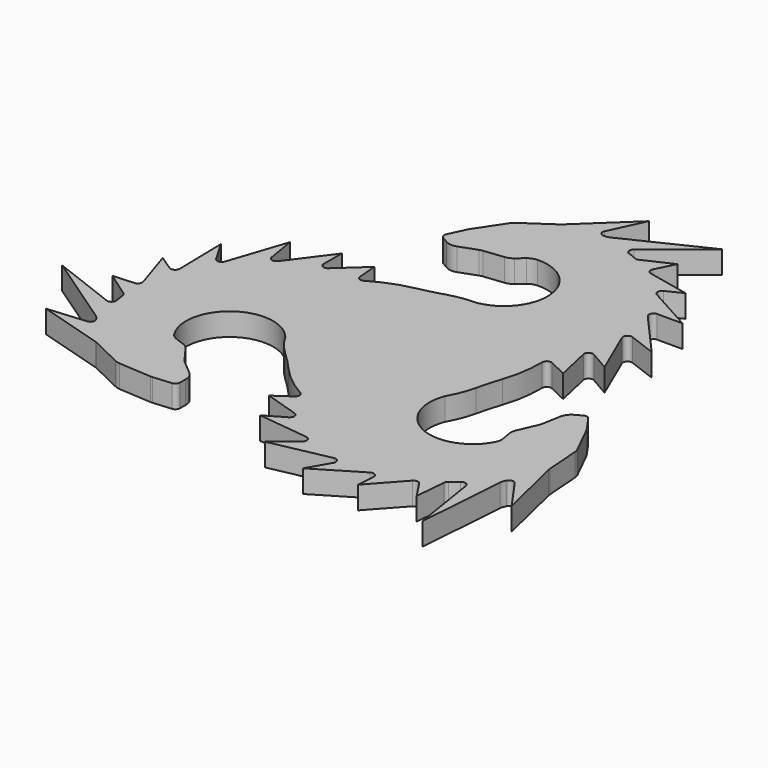
from build123d import *

# Parameters (mm, degrees)
F0_R     = 14.2772692689
F1_DEPTH = 5
F2_R     = 55
F3_R     = 1
F4_R     = 1
F5_COUNT = 3
F7_R     = 14.2772692689
F8_DEPTH = 5


# Not quite as in the source:
# - a feature names something its author has since deleted; it is built from what else it names


with BuildPart() as f1:
    # F0 (on Top) → F1 (new body)
    with BuildSketch(Plane.XY):
        with BuildLine():
            ThreePointArc((20.3165472355, -1.8543326892), (20.3798729378, -0.9281273257), (20.4009960858, 0))
            ThreePointArc((20.4009960858, 0), (20.0666164726, 3.6785247903), (19.0744388358, 7.23646491))
            ThreePointArc((19.0744388358, 7.23646491), (11.5881307593, 16.7903504072), (0, 20.4009960858))
            ThreePointArc((0, 20.4009960858), (-15.0670314798, -13.7544612282), (20.3165472355, -1.8543326892))
        make_face()
        Circle(F0_R, mode=Mode.SUBTRACT)
        with BuildLine():
            ThreePointArc((19.0744388358, 7.23646491), (20.0666164726, 3.6785247903), (20.4009960858, 0))
            ThreePointArc((20.4009960858, 0), (20.3798729378, -0.9281273257), (20.3165472355, -1.8543326892))
            ThreePointArc((20.3165472355, -1.8543326892), (22.4085751719, 4.7991946551), (22.7576271971, 11.7651238603))
            ThreePointArc((22.7576271971, 11.7651238603), (21.0408953007, 9.3992430611), (19.0744388358, 7.23646491))
        make_face()
        with BuildLine():
            ThreePointArc((0, 20.4009960858), (11.5881307593, 16.7903504072), (19.0744388358, 7.23646491))
            ThreePointArc((19.0744388358, 7.23646491), (21.0408953007, 9.3992430611), (22.7576271971, 11.7651238603))
            ThreePointArc((22.7576271971, 11.7651238603), (24.6772177681, 15.306857196), (26.0387565941, 19.0982837094))
            ThreePointArc((26.0387565941, 19.0982837094), (26.862971826, 23.5334397962), (26.9242947963, 28.0441137764))
            ThreePointArc((26.9242947963, 28.0441137764), (26.2417321911, 32.4151242488), (24.8427105993, 36.6120710969))
            ThreePointArc((24.8427105993, 36.6120710969), (23.0649012349, 40.043318935), (20.8077298225, 43.1800760308))
            ThreePointArc((20.8077298225, 43.1800760308), (18.3116216059, 45.7823431307), (15.485866915, 48.02231204))
            ThreePointArc((15.485866915, 48.02231204), (13.5514525795, 49.2332070536), (11.520179105, 50.2734731867))
            ThreePointArc((11.520179105, 50.2734731867), (9.4992839441, 51.1021592503), (7.4171009474, 51.7618954182))
            Line((7.4171009474, 51.7618954182), (20.6731967628, 62.493018806))
            Line((20.6731967628, 62.493018806), (2.9851620813, 53.9539658583))
            ThreePointArc((2.9851620813, 53.9539658583), (2.3498823759, 53.7311579429), (1.6809146705, 53.6556206644))
            Line((1.6809146705, 53.6556206644), (0, 53.6556206644))
            Line((0, 53.6556206644), (4.2608887888, 62.8086403012))
            Line((4.2608887888, 62.8086403012), (-6.6135251858, 52.5556231266))
            ThreePointArc((-6.6135251858, 52.5556231266), (-6.7917072446, 52.4004137483), (-6.9815525166, 52.2597099106))
            Line((-6.9815525166, 52.2597099106), (-13.2472028108, 47.9876733272))
            ThreePointArc((-13.2472028108, 47.9876733272), (-13.6895314092, 47.6192351761), (-14.0533422232, 47.1730928761))
            Line((-14.0533422232, 47.1730928761), (-18.0220315222, 41.2200618552))
            ThreePointArc((-18.0220315222, 41.2200618552), (-18.1407171431, 41.0265497088), (-18.2444304369, 40.824617096))
            Line((-18.2444304369, 40.824617096), (-20.3575752676, 36.2964496017))
            Line((-20.3575752676, 36.2964496017), (-18.2173253559, 35.0123005809))
            ThreePointArc((-18.2173253559, 35.0123005809), (-16.9608718875, 34.5985427406), (-15.6486105692, 34.7653992696))
            Line((-15.6486105692, 34.7653992696), (-11.8852458251, 36.1338942554))
            ThreePointArc((-11.8852458251, 36.1338942554), (-11.5431146027, 36.2357083507), (-11.1913122519, 36.2961648589))
            Line((-11.1913122519, 36.2961648589), (-6.7715043443, 36.7872549082))
            ThreePointArc((-6.7715043443, 36.7872549082), (-5.920047927, 37.0118969078), (-5.1704976221, 37.4740834492))
            Line((-5.1704976221, 37.4740834492), (-3.5822876233, 38.8113983631))
            ThreePointArc((-3.5822876233, 38.8113983631), (-2.7243104061, 39.3176161279), (-1.7478732612, 39.5149783142))
            ThreePointArc((-1.7478732612, 39.5149783142), (8.1392001596, 30.7821912097), (0, 20.4009960858))
        make_face()
        with BuildLine():
            ThreePointArc((26.0387565941, 19.0982837094), (24.6772177681, 15.306857196), (22.7576271971, 11.7651238603))
            Line((22.7576271971, 11.7651238603), (28.2481051981, 9.1530177742))
            Line((28.2481051981, 9.1530177742), (26.0387565941, 19.0982837094))
        make_face()
        with BuildLine():
            ThreePointArc((26.9242947963, 28.0441137764), (26.862971826, 23.5334397962), (26.0387565941, 19.0982837094))
            Line((26.0387565941, 19.0982837094), (32.3511809111, 15.4654439539))
            Line((32.3511809111, 15.4654439539), (26.9242947963, 28.0441137764))
        make_face()
        with BuildLine():
            ThreePointArc((24.8427105993, 36.6120710969), (26.2417321911, 32.4151242488), (26.9242947963, 28.0441137764))
            Line((26.9242947963, 28.0441137764), (35.1917743683, 24.9340832233))
            Line((35.1917743683, 24.9340832233), (24.8427105993, 36.6120710969))
        make_face()
        with BuildLine():
            ThreePointArc((20.8077298225, 43.1800760308), (23.0649012349, 40.043318935), (24.8427105993, 36.6120710969))
            Line((24.8427105993, 36.6120710969), (32.6668024063, 36.6120710969))
            Line((32.6668024063, 36.6120710969), (20.8077298225, 43.1800760308))
        make_face()
        with BuildLine():
            ThreePointArc((15.485866915, 48.02231204), (18.3116216059, 45.7823431307), (20.8077298225, 43.1800760308))
            Line((20.8077298225, 43.1800760308), (26.0387565941, 45.7650870085))
            Line((26.0387565941, 45.7650870085), (15.485866915, 48.02231204))
        make_face()
        with BuildLine():
            ThreePointArc((11.520179105, 50.2734731867), (13.5514525795, 49.2332070536), (15.485866915, 48.02231204))
            Line((15.485866915, 48.02231204), (18.1482266635, 53.3400028944))
            Line((18.1482266635, 53.3400028944), (11.520179105, 50.2734731867))
        make_face()
    extrude(amount=F1_DEPTH)

    # F2
    f2_edges = [f1.edges().sort_by_distance(p)[0] for p in [
        (20.316547, -1.854333, 2.5),
    ]]
    fillet(f2_edges, radius=F2_R)

    # F3
    f3_edges = [f1.edges().sort_by_distance(p)[0] for p in [
        (22.757627, 11.765124, 2.5),
        (26.038757, 19.098284, 2.5),
        (26.924295, 28.044114, 2.5),
        (24.842711, 36.612071, 2.5),
        (20.80773, 43.180076, 2.5),
        (15.485867, 48.022312, 2.5),
        (11.520179, 50.273473, 2.5),
        (7.417101, 51.761895, 2.5),
        (0, 53.655621, 2.5),
    ]]
    fillet(f3_edges, radius=F3_R)

    # F4
    f4_edges = [f1.edges().sort_by_distance(p)[0] for p in [
        (-20.357575, 36.29645, 2.5),
    ]]
    fillet(f4_edges, radius=F4_R)


with BuildPart() as f5_1:
    # F5: instance of F1
    add(f1.part.rotate(Axis((0, 0, 5), (0, 0, 1)), 1 * 360 / F5_COUNT))


with BuildPart() as f5_2:
    # F5: instance of F1
    add(f1.part.rotate(Axis((0, 0, 5), (0, 0, 1)), 2 * 360 / F5_COUNT))


with BuildPart() as f1_1:
    add(f1.part)

    # F6: union 

    add(f5_1.part)  # F8 merges F5_1

    add(f5_2.part)  # F8 merges F5_2
    # F7 (on face) → F8 (join)
    with BuildSketch(Plane.XY.offset(5)):
        Circle(F7_R)
    extrude(amount=-F8_DEPTH)


solid = f1_1.part
